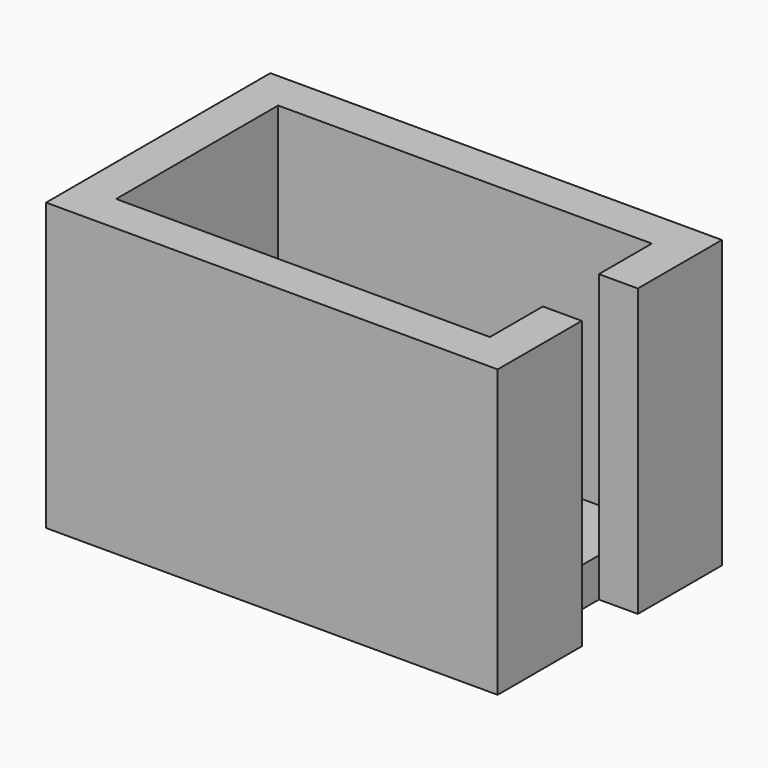
from build123d import *

# Parameters (mm, degrees)
F0_W     = 24
F0_H     = 13
F1_DEPTH = 15.9
F2_T     = 2.5
F3_W     = 4.5
F3_H     = 2.5
F4_DEPTH = 2.5


with BuildPart() as f1:
    # F0 (on Top) → F1 (new body)
    with BuildSketch(Plane.XY):
        with Locations((-7.2094501108, -16.6747012585)):
            Rectangle(F0_W, F0_H)
    extrude(amount=-F1_DEPTH)

    # F2
    f2_openings = [f1.faces().sort_by_distance(p)[0] for p in [
        (-7.20945, -16.674701, 0),
    ]]
    offset(amount=F2_T, openings=f2_openings, kind=Kind.INTERSECTION)

    # F3 (on face) → F4 (cut)
    with BuildSketch(Plane.YZ.offset(7.2905498892)):
        Polygon((-14.4247012585, 0), (-16.6747012585, 0), (-18.9247012585, 0), (-18.9247012585, -15.9), (-14.4247012585, -15.9), align=None)
        with Locations((-16.6747012585, -17.15)):
            Rectangle(F3_W, F3_H)
    extrude(amount=-F4_DEPTH, mode=Mode.SUBTRACT)


solid = f1.part
